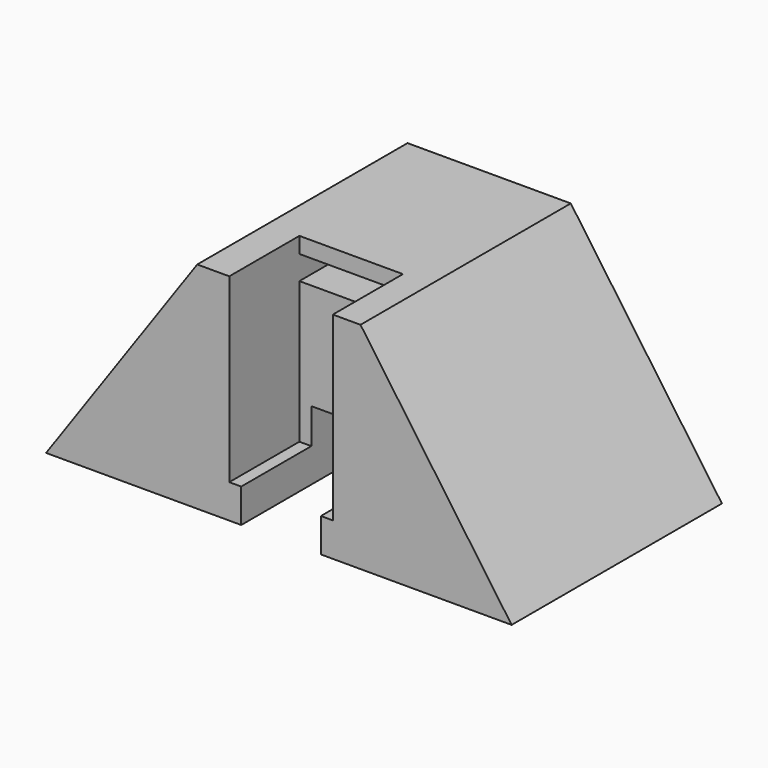
from build123d import *

# Parameters (mm, degrees)
F1_DEPTH = 33
F2_W     = 13
F2_H     = 22.75
F3_DEPTH = 11
F4_W     = 13
F4_H     = 3
F5_DEPTH = 5


# Not quite as in the source:
# - a feature of the source that left no trace in its solid (it failed there, or was rolled back) is left out


with BuildPart() as f1:
    # F0 (on Front) → F1 (new body)
    with BuildSketch(Plane.XZ):
        Polygon((-10.526334039, 27), (-29.5, 0), (-5, 0), (-5, 8.67), (5, 8.67), (5, 0), (28.947331922, 0), (9.973665961, 27), align=None)
    extrude(amount=F1_DEPTH)

    # F2 (on face) → F3 (cut)
    with BuildSketch(Plane.XZ.offset(33)):
        with Locations((0, 15.625)):
            Rectangle(F2_W, F2_H)
    extrude(amount=-F3_DEPTH, mode=Mode.SUBTRACT)

    # F4 (on face) → F5 (cut)
    with BuildSketch(Plane.XZ.offset(22)):
        with Locations((0, 23.5)):
            Rectangle(F4_W, F4_H)
    extrude(amount=-F5_DEPTH, mode=Mode.SUBTRACT)


solid = f1.part
